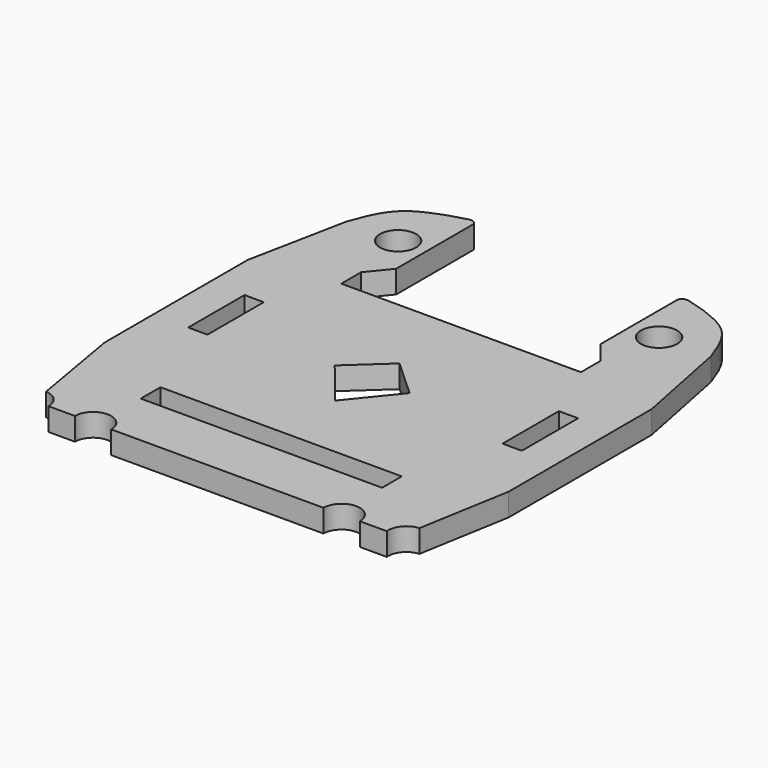
from build123d import *

# Parameters (mm, degrees)
F0_R     = 1.6
F1_DEPTH = 2


# Not quite as in the source:
# - ends of sketch curves that miss each other by under 0.0002 mm in the source are joined


with BuildPart() as f1:
    # F0 (on Top) → F1 (new body)
    with BuildSketch(Plane.XY):
        with BuildLine():
            ThreePointArc((9.4743104318, 0.2374556452), (11.0743104318, 1.8374556452), (12.6743104318, 0.2374556452))
            Line((12.6743104318, 0.2374556452), (22.0509076786, 0.2374556452))
            Line((22.0509076786, 0.2374556452), (31.3863246398, 0.2374556452))
            ThreePointArc((31.3863246398, 0.2374556452), (32.9863104318, 1.8374556452), (34.5863104318, 0.2374556452))
            Line((34.5863104318, 0.2374556452), (36.9589188956, 0.2374556452))
            ThreePointArc((36.9589188956, 0.2374556452), (37.322944486, 1.4299580557), (38.4322782501, 1.9991287063))
            Line((38.4322782501, 1.9991287063), (39.8303104318, 10.0774704438))
            Line((39.8303104318, 10.0774704438), (39.8303104318, 25.8181473703))
            Line((39.8303104318, 25.8181473703), (38.0968938881, 34.5188772837))
            add(Edge.make_bspline(
                [(38.0968938881, 34.5188772837), (37.6683242364, 35.7597207754), (36.7252101224, 38.130874007), (34.7779775897, 39.0193902227), (33.5303104318, 39.4987425759)],
                knots=[0, 0, 0, 0, 0.51039131, 1, 1, 1, 1], degree=3))
            ThreePointArc((33.5303104318, 39.4987425759), (32.6165966127, 39.7845023129), (31.6957953827, 40.0465264824))
            ThreePointArc((31.6957953827, 40.0465264824), (31.3007464304, 40.007865889), (31.0303104318, 39.7173100649))
            Line((31.0303104318, 39.7173100649), (31.0303104318, 34.5188772837))
            Line((31.0303104318, 34.5188772837), (31.0303104318, 31.1867967248))
            Line((31.0303104318, 31.1867967248), (32.5903408229, 29.2609930038))
            Line((32.5903408229, 29.2609930038), (32.5903408229, 27.0907320082))
            Line((32.5903408229, 27.0907320082), (22.0303104318, 27.0907320082))
            Line((22.0303104318, 27.0907320082), (11.4702800406, 27.0907320082))
            Line((11.4702800406, 27.0907320082), (11.4702800406, 29.2609930038))
            Line((11.4702800406, 29.2609930038), (13.0303104318, 31.1867967248))
            Line((13.0303104318, 31.1867967248), (13.0303104318, 34.5188772837))
            Line((13.0303104318, 34.5188772837), (13.0303104318, 39.7173100649))
            ThreePointArc((13.0303104318, 39.7173100649), (12.7598744332, 40.007865889), (12.3648254809, 40.0465264824))
            ThreePointArc((12.3648254809, 40.0465264824), (11.4440242509, 39.7845023129), (10.5303104318, 39.4987425759))
            add(Edge.make_bspline(
                [(5.9637269754, 34.5188772837), (6.3922966272, 35.7597207754), (7.3354107411, 38.130874007), (9.2826432739, 39.0193902227), (10.5303104318, 39.4987425759)],
                knots=[0, 0, 0, 0, 0.51039131, 1, 1, 1, 1], degree=3))
            Line((5.9637269754, 34.5188772837), (4.2303104318, 25.8181473703))
            Line((4.2303104318, 25.8181473703), (4.2303104318, 10.0774704438))
            Line((4.2303104318, 10.0774704438), (5.6569326528, 1.8339249926))
            ThreePointArc((5.6569326528, 1.8339249926), (6.7190254428, 1.3306221238), (7.1506988404, 0.2374556452))
            Line((7.1506988404, 0.2374556452), (9.4743104318, 0.2374556452))
        make_face()
        Polygon((11.5445189413, 7.2601027762), (22.0303104318, 7.2601027762), (32.5161019223, 7.2601027762), (32.6645797236, 7.2601027762), (32.6645797236, 5.0898417806), (32.5161019223, 5.0898417806), (11.5445189413, 5.0898417806), (11.39604114, 5.0898417806), (11.39604114, 7.2601027762), align=None, mode=Mode.SUBTRACT)
        Polygon((18.7320070459, 17.286), (22.0303104318, 20.3086156398), (25.3286138177, 17.286), (22.0303104318, 13.222059235), align=None, mode=Mode.SUBTRACT)
        Polygon((8.1803104318, 15.401), (7.3303104318, 15.401), (7.3303104318, 21.601), (8.1803104318, 21.601), (9.0303104318, 21.601), (9.0303104318, 15.401), align=None, mode=Mode.SUBTRACT)
        with Locations((10.5303104318, 34.5188772837)):
            Circle(F0_R, mode=Mode.SUBTRACT)
        Polygon((35.0303104318, 15.401), (35.0303104318, 21.601), (35.8803104318, 21.601), (36.7303104318, 21.601), (36.7303104318, 15.401), (35.8803104318, 15.401), align=None, mode=Mode.SUBTRACT)
        with Locations((33.5303104318, 34.5188772837)):
            Circle(F0_R, mode=Mode.SUBTRACT)
    extrude(amount=F1_DEPTH)


solid = f1.part
